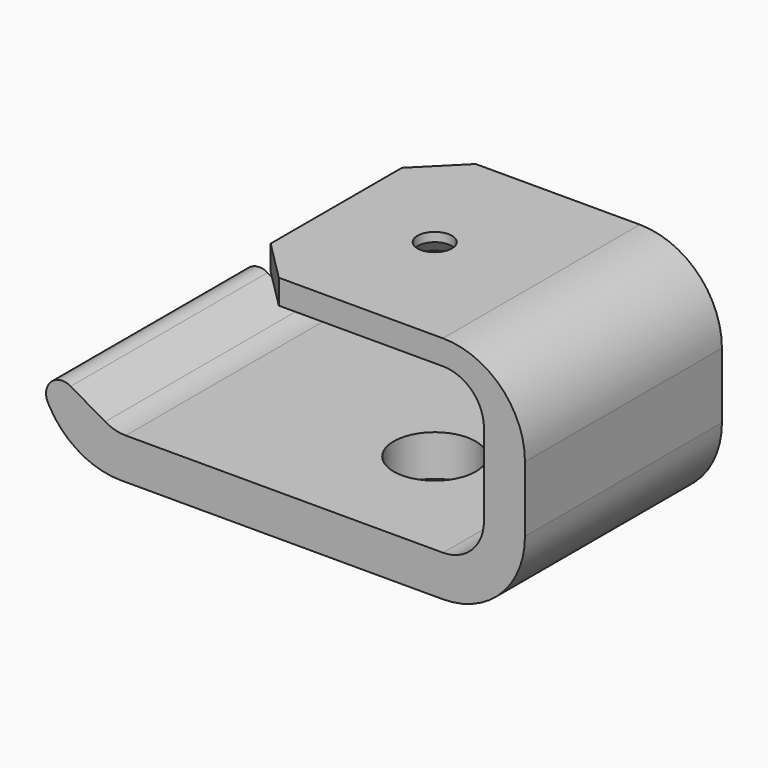
from build123d import *

# Parameters (mm, degrees)
F1_DEPTH       = 15
F2_R           = 5
F3_R           = 10
F5_D           = 4.2
F5_CSINK_D     = 8
F5_CSINK_ANGLE = 90
F6_R           = 5
F7_DEPTH       = 5
F8_T1_DEPTH    = 47.7203429425
F9_R           = 2
F10_SIZE       = 5


# Not quite as in the source:
# - a fillet or chamfer that OpenCascade refuses, or shapes differently, is made with other operations: its cross-section is extruded or revolved along the edge and cut away or added


with BuildPart() as f1:
    # F0 (on Front) → F1 (new body, symmetric)
    with BuildSketch(Plane.XZ):
        Polygon((0, 3), (0, 0), (30, 0), (30, -20), (-15, -20), (-23.6602540378, -15), (-25.0838401426, -16.1945305755), (-20, -25), (35, -25), (35, 3), align=None)
    extrude(amount=F1_DEPTH, both=True)

    # F2
    f2_edges = [f1.edges().sort_by_distance(p)[0] for p in [
        (30, 0, 0),
        (30, 0, -20),
        (-15, 0, -20),
    ]]
    fillet(f2_edges, radius=F2_R)

    # F3
    f3_edges = [f1.edges().sort_by_distance(p)[0] for p in [
        (35, 0, 3),
        (35, 0, -25),
        (-20, 0, -25),
    ]]
    fillet(f3_edges, radius=F3_R)

    # F5 (through all)
    with Locations(Plane(origin=(0, 0, 0), x_dir=(1, 0, 0), z_dir=(0, 0, -1))):
        with Locations((12, 0)):
            CounterSinkHole(F5_D / 2, F5_CSINK_D / 2, counter_sink_angle=F5_CSINK_ANGLE)

    # F6 (on face) → F7 (cut, through all)
    with BuildSketch(Plane(origin=(0, 0, -25), x_dir=(1, 0, 0), z_dir=(0, 0, -1))):
        with Locations((12, 0)):
            Circle(F6_R)
    extrude(amount=-F7_DEPTH, mode=Mode.SUBTRACT)

    # F8: fillet of radius 5 on 1 edges, made by hand

    # F8_s2 → F8_t1 (cut)
    with BuildSketch(Plane.XZ.offset(-23.8601714713)):
        with BuildLine():
            ThreePointArc((-23.3118058484, -19.2637840059), (-23.9650654758, -17.171040108), (-23.6602540378, -15))
            Line((-23.6602540378, -15), (-25.0838401426, -16.1945305755))
            Line((-25.0838401426, -16.1945305755), (-23.3118058484, -19.2637840059))
        make_face()
    extrude(amount=F8_T1_DEPTH, mode=Mode.SUBTRACT)

    # F9
    f9_edges = [f1.edges().sort_by_distance(p)[0] for p in [
        (-23.660254, 0, -15),
    ]]
    fillet(f9_edges, radius=F9_R)

    # F10
    f10_edges = [f1.edges().sort_by_distance(p)[0] for p in [
        (0, 15, 1.5),
        (0, -15, 1.5),
    ]]
    chamfer(f10_edges, length=F10_SIZE)


solid = f1.part
